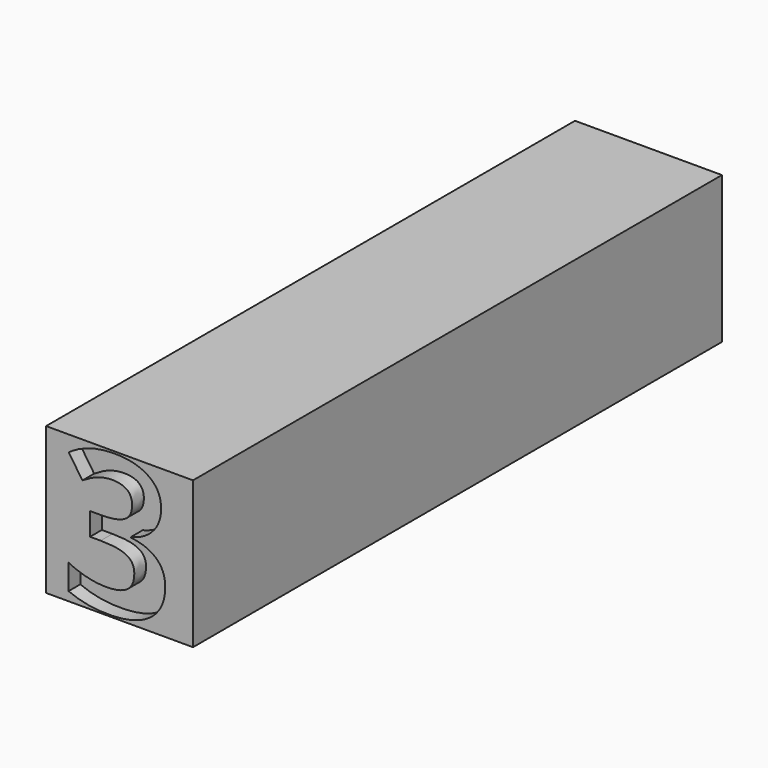
from build123d import *

# Parameters (mm, degrees)
F0_W         = 25.4
F0_H         = 25.4
F1_DEPTH     = 114.3
F2_TEXT_SIZE = 33.8264765257
F3_DEPTH     = 2.54


# Not quite as in the source:
# - Text() gives the source's letters only with a copy of the font that has no kerning and outlines rounded to 1/6400 em; it was checked with that copy


with BuildPart() as f1:
    # F0 (on Front) → F1 (new body)
    with BuildSketch(Plane.XZ):
        with Locations((12.7, 12.7)):
            Rectangle(F0_W, F0_H)
    extrude(amount=F1_DEPTH)

    # F2 (on face) → F3 (cut)
    with BuildSketch(Plane.XZ.offset(114.3)):
        with Locations((2.5962658692, 0.5706959637)):
            Text('3', F2_TEXT_SIZE, font='Open Sans', font_style=FontStyle.BOLD, text_align=(TextAlign.LEFT, TextAlign.BOTTOM))
    extrude(amount=-F3_DEPTH, mode=Mode.SUBTRACT)


solid = f1.part
